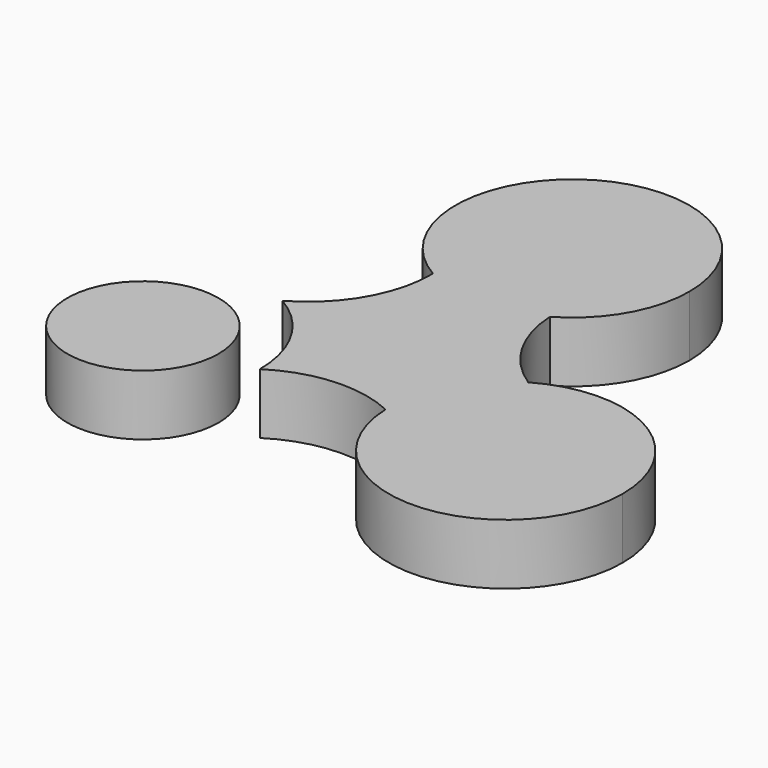
from build123d import *

# Parameters (mm, degrees)
F0_R     = 11.0871
F1_DEPTH = 8.89


# Not quite as in the source:
# - a feature names something its author has since deleted; it is built from what else it names


with BuildPart() as f1:
    # F0 (on Top) → F1 (new body)
    with BuildSketch(Plane.XY):
        with BuildLine():
            ThreePointArc((16.7904205794, 1.398138476), (10.362351598, -5.1472195886), (8.22912946, -14.0697274387))
            ThreePointArc((8.22912946, -14.0697274387), (25.672901431, -30.5920646228), (42.5079205794, -13.4498670719))
            ThreePointArc((42.5079205794, -13.4498670719), (33.9354205794, 1.398138476), (16.7904205794, 1.398138476))
        make_face()
        with Locations((25.3629205794, -13.4498670719)):
            Circle(F0_R, mode=Mode.SUBTRACT)
        with BuildLine():
            ThreePointArc((17.145, 30.48), (-8.5725, 45.3280055479), (-8.5725, 15.6319944521))
            ThreePointArc((-8.5725, 15.6319944521), (0, 13.335), (8.5725, 15.6319944521))
            ThreePointArc((8.5725, 15.6319944521), (14.8480055479, 21.9075), (17.145, 30.48))
        make_face()
        with Locations((0, 30.48)):
            Circle(F0_R, mode=Mode.SUBTRACT)
        with BuildLine():
            ThreePointArc((-17.8239543073, -0.3919944521), (-11.5484487595, -6.6675), (-9.2514543073, -15.24))
            ThreePointArc((-9.2514543073, -15.24), (-0.6623230767, -12.3969483031), (8.22912946, -14.0697274387))
            ThreePointArc((8.22912946, -14.0697274387), (10.362351598, -5.1472195886), (16.7904205794, 1.398138476))
            ThreePointArc((16.7904205794, 1.398138476), (10.971190185, 7.5276415587), (8.5725, 15.6319944521))
            ThreePointArc((8.5725, 15.6319944521), (0, 13.335), (-8.5725, 15.6319944521))
            ThreePointArc((-8.5725, 15.6319944521), (-10.9939497148, 6.3473598273), (-17.8239543073, -0.3919944521))
        make_face()
        Circle(F0_R, mode=Mode.SUBTRACT)
        Circle(F0_R)
        with Locations((0, 30.48)):
            Circle(F0_R)
        with Locations((25.3629205794, -13.4498670719)):
            Circle(F0_R)
    extrude(amount=F1_DEPTH)


with BuildPart() as f1b:
    # F0 (on Top) → F1, piece 2 (new body)
    with BuildSketch(Plane.XY):
        with Locations((-26.3964543073, -15.24)):
            Circle(F0_R)
    extrude(amount=F1_DEPTH)


solid = Compound([f1.part, f1b.part])
